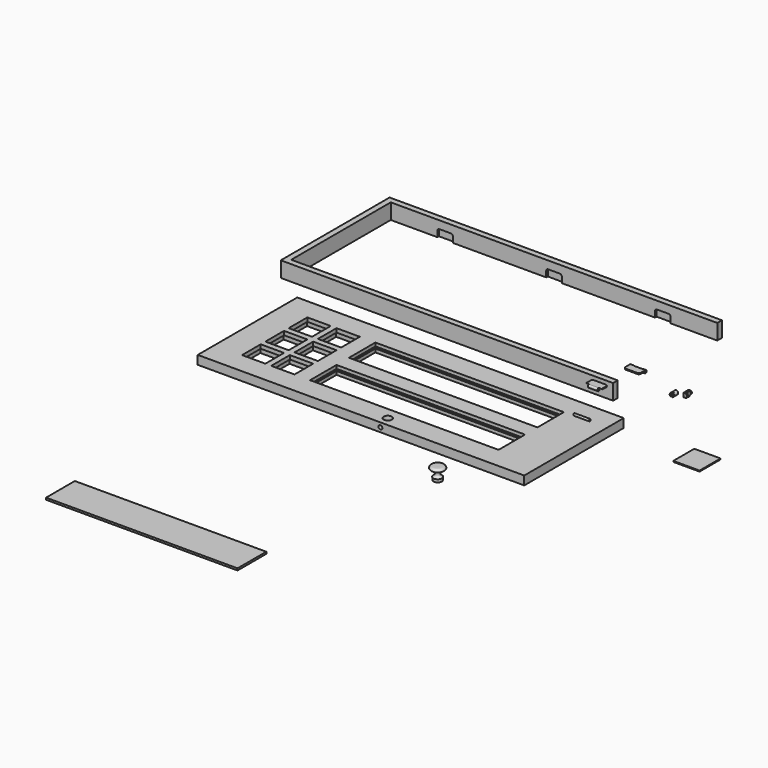
from build123d import *

# Parameters (mm, degrees)
F0_W      = 2133.6
F0_H      = 812.8
F0_W_2    = 152.4
F0_H_2    = 152.4
F0_W_3    = 1231.9
F0_H_3    = 215.9
F1_DEPTH  = 57.15
F2_R      = 6.985
F3_DEPTH  = 101.6
F6_DEPTH  = 63.5
F8_DEPTH  = 101.6
F10_R     = 9.525
F10_R_2   = 6.985
F11_DEPTH = 31.75
F12_R     = 6.985
F13_DEPTH = 101.6
F14_R     = 12.7
F14_2_R   = 12.7
F15_W     = 101.6
F15_H     = 50.8
F16_DEPTH = 6.35
F17_R     = 12.7
F19_DEPTH = 101.6
F20_W     = 101.6
F20_H     = 50.8
F21_DEPTH = 12.7
F22_R     = 12.7
F23_R     = 26.9875
F24_DEPTH = 393.7
F26_DEPTH = 57.658
F29_W     = 1250.95
F29_H     = 234.95
F29_W_2   = 1231.9
F29_H_2   = 215.9
F32_DEPTH = 12.7
F31_W     = 2.4516191959
F31_H     = 12.7
F31_W_2   = 9.525
F34_W     = 9.525
F34_H     = 12.7
F36_W     = 171.45
F36_H     = 171.45
F36_W_2   = 152.4
F36_H_2   = 152.4
F37_DEPTH = 31.75
F38_W     = 171.45
F38_H     = 171.45
F39_DEPTH = 6.35
F40_R     = 12.7
F41_DEPTH = 38.1
F42_W     = 12.7
F42_H     = 49.1664424331
F43_DEPTH = 12.7
F45_DEPTH = 39.624
F46_W     = 12.7
F46_H     = 25.4
F47_DEPTH = 50.8
F49_R     = 3.81
F50_DEPTH = 12.7
F51_R     = 12.69999
F52_W     = 9.8214453638
F52_H     = 25.4
F53_DEPTH = 6.35
F55_DEPTH = 12.7
F56_R     = 26.9875
F57_DEPTH = 19.05
F59_DEPTH = 12.7


# Not quite as in the source:
# - a fillet or chamfer is up to 0.001 mm smaller than in the source, because OpenCascade refuses the exact size


with BuildPart() as f1:
    # F0 (on Top) → F1 (new body)
    with BuildSketch(Plane.XY):
        with Locations((-1066.8, -406.4)):
            Rectangle(F0_W, F0_H)
        with Locations((-1879.6, -596.9)):
            Rectangle(F0_W_2, F0_H_2, mode=Mode.SUBTRACT)
        with Locations((-1689.1, -596.9)):
            Rectangle(F0_W_2, F0_H_2, mode=Mode.SUBTRACT)
        with Locations((-1879.6, -406.4)):
            Rectangle(F0_W_2, F0_H_2, mode=Mode.SUBTRACT)
        with Locations((-1689.1, -406.4)):
            Rectangle(F0_W_2, F0_H_2, mode=Mode.SUBTRACT)
        with Locations((-895.35, -565.15)):
            Rectangle(F0_W_3, F0_H_3, mode=Mode.SUBTRACT)
        with Locations((-1879.6, -215.9)):
            Rectangle(F0_W_2, F0_H_2, mode=Mode.SUBTRACT)
        with Locations((-1689.1, -215.9)):
            Rectangle(F0_W_2, F0_H_2, mode=Mode.SUBTRACT)
        with Locations((-895.35, -247.65)):
            Rectangle(F0_W_3, F0_H_3, mode=Mode.SUBTRACT)
    extrude(amount=F1_DEPTH)

    # F15 (on face) → F16 (cut)
    with BuildSketch(Plane(origin=(0, 0, 0), x_dir=(-1, 0, 0), z_dir=(0, 1, 0))):
        with Locations((355.6, 25.4)):
            Rectangle(F15_W, F15_H)
        with Locations((1778, 25.4)):
            Rectangle(F15_W, F15_H)
        with Locations((1066.8, 25.4)):
            Rectangle(F15_W, F15_H)
    extrude(amount=-F16_DEPTH, mode=Mode.SUBTRACT)

    # F17
    f17_edges = [f1.edges().sort_by_distance(p)[0] for p in [
        (-304.8, -3.175, 50.8),
        (-406.4, -3.175, 50.8),
        (-1117.6, -3.175, 50.8),
        (-1016, -3.175, 50.8),
        (-1727.2, -3.175, 50.8),
        (-1828.8, -3.175, 50.8),
    ]]
    fillet(f17_edges, radius=F17_R)

    # F23 (on face) → F24 (cut)
    with BuildSketch(Plane(origin=(0, 0, 0), x_dir=(1, 0, 0), z_dir=(0, 0, -1))):
        with Locations((-939.8, 752.475)):
            Circle(F23_R)
    extrude(amount=-F24_DEPTH, mode=Mode.SUBTRACT)

    # F25 (on face) → F26 (cut)
    with BuildSketch(Plane.XZ.offset(812.8)):
        with BuildLine():
            ThreePointArc((-952.5, 28.575), (-939.8, 15.875), (-927.1, 28.575))
            Line((-927.1, 28.575), (-952.5, 28.575))
        make_face()
        with BuildLine():
            Line((-952.5, 28.575), (-927.1, 28.575))
            ThreePointArc((-927.1, 28.575), (-939.8, 41.275), (-952.5, 28.575))
        make_face()
    extrude(amount=-F26_DEPTH, mode=Mode.SUBTRACT)

    # F33: sweep along a path in F33_path
    with BuildLine(Plane(origin=(-1511.3, -457.2, 0), x_dir=(0, 1, 0), z_dir=(0, 0, 1))) as f33_path:
        Line((0, 0), (0, -1231.9))
        Line((0, -1231.9), (-215.9, -1231.9))
        Line((-215.9, -1231.9), (-215.9, 0))
        Line((-215.9, 0), (0, 0))
    # F31 (on offset) → F33 (sweep, cut)
    with BuildSketch(Plane.YZ.offset(-627.38)):
        with Locations((-458.425809598, 28.575)):
            Rectangle(F31_W, F31_H)
        with Locations((-452.4375, 28.575)):
            Rectangle(F31_W_2, F31_H)
    sweep(path=f33_path.line, transition=Transition.RIGHT, mode=Mode.SUBTRACT)

    # F35: sweep along a path in F35_path
    with BuildLine(Plane(origin=(-279.4, -355.6, 0), x_dir=(0, 1, 0), z_dir=(0, 0, 1))) as f35_path:
        Line((0, 0), (0, 1231.9))
        Line((0, 1231.9), (215.9, 1231.9))
        Line((215.9, 1231.9), (215.9, 0))
        Line((215.9, 0), (0, 0))
    # F34 (on offset) → F35 (sweep, cut)
    with BuildSketch(Plane.YZ.offset(-627.38)):
        with Locations((-360.3625, 28.575)):
            Rectangle(F34_W, F34_H)
    sweep(path=f35_path.line, transition=Transition.RIGHT, mode=Mode.SUBTRACT)

    # F36 (on face) → F37 (cut)
    with BuildSketch(Plane(origin=(0, 0, 0), x_dir=(1, 0, 0), z_dir=(0, 0, -1))):
        with Locations((-1689.1, 596.9)):
            Rectangle(F36_W, F36_H)
        with Locations((-1689.1, 596.9)):
            Rectangle(F36_W_2, F36_H_2, mode=Mode.SUBTRACT)
        with Locations((-1879.6, 596.9)):
            Rectangle(F36_W, F36_H)
        with Locations((-1879.6, 596.9)):
            Rectangle(F36_W_2, F36_H_2, mode=Mode.SUBTRACT)
        with Locations((-1879.6, 406.4)):
            Rectangle(F36_W, F36_H)
        with Locations((-1879.6, 406.4)):
            Rectangle(F36_W_2, F36_H_2, mode=Mode.SUBTRACT)
        with Locations((-1689.1, 406.4)):
            Rectangle(F36_W, F36_H)
        with Locations((-1689.1, 406.4)):
            Rectangle(F36_W_2, F36_H_2, mode=Mode.SUBTRACT)
        with Locations((-1689.1, 215.9)):
            Rectangle(F36_W, F36_H)
        with Locations((-1689.1, 215.9)):
            Rectangle(F36_W_2, F36_H_2, mode=Mode.SUBTRACT)
        with Locations((-1879.6, 215.9)):
            Rectangle(F36_W, F36_H)
        with Locations((-1879.6, 215.9)):
            Rectangle(F36_W_2, F36_H_2, mode=Mode.SUBTRACT)
    extrude(amount=-F37_DEPTH, mode=Mode.SUBTRACT)


with BuildPart() as f3:
    # F2 (on Right) → F3 (new body)
    with BuildSketch(Plane.YZ):
        with BuildLine():
            Line((0, 339.3088579178), (41.8197438789, 339.3088579178))
            ThreePointArc((41.8197438789, 339.3088579178), (56.299261314, 328.3567279844), (50.8, 345.6588579178))
            Line((50.8, 345.6588579178), (0, 345.6588579178))
            Line((0, 345.6588579178), (0, 339.3088579178))
        make_face()
        with Locations((50.8, 336.1338579178)):
            Circle(F2_R, mode=Mode.SUBTRACT)
    extrude(amount=F3_DEPTH)

    # F5 (on offset) → F6 (cut)
    with BuildSketch(Plane.YZ.offset(82.55)):
        with BuildLine():
            ThreePointArc((50.8, 345.6588579178), (44.0648079092, 329.398665827), (60.325, 336.1338579178))
            ThreePointArc((60.325, 336.1338579178), (57.5351920908, 342.8690500086), (50.8, 345.6588579178))
        make_face()
    extrude(amount=-F6_DEPTH, mode=Mode.SUBTRACT)

    # F14#2
    f14_2_edges = [f3.edges().sort_by_distance(p)[0] for p in [
        (101.6, 0, 342.483858),
        (0, 0, 342.483858),
    ]]
    fillet(f14_2_edges, radius=F14_2_R)


with BuildPart() as f8:
    # F7 (on Right) → F8 (new body)
    with BuildSketch(Plane.YZ):
        with BuildLine():
            ThreePointArc((-181.1577074063, 298.6267453909), (-175.6584460923, 296.8788753242), (-172.1774512852, 292.2767453909))
            Line((-172.1774512852, 292.2767453909), (-130.3577074063, 292.2767453909))
            Line((-130.3577074063, 292.2767453909), (-130.3577074063, 298.6267453909))
            Line((-130.3577074063, 298.6267453909), (-181.1577074063, 298.6267453909))
        make_face()
    extrude(amount=-F8_DEPTH)

    # F10 (on offset) → F11 (join, symmetric)
    with BuildSketch(Plane.YZ.offset(-50.8)):
        with Locations((-181.1577074063, 289.1017453909)):
            Circle(F10_R)
        with Locations((-181.1577074063, 289.1017453909)):
            Circle(F10_R_2, mode=Mode.SUBTRACT)
    extrude(amount=F11_DEPTH, both=True)

    # F14
    f14_edges = [f8.edges().sort_by_distance(p)[0] for p in [
        (0, -130.357707, 295.451745),
        (-101.6, -130.357707, 295.451745),
    ]]
    fillet(f14_edges, radius=F14_R)


with BuildPart() as f13:
    # F12 (on Right) → F13 (new body)
    with BuildSketch(Plane.YZ):
        with Locations((-277.2486507893, 157.7363908291)):
            Circle(F12_R)
    extrude(amount=-F13_DEPTH)


with BuildPart() as f19:
    # F18 (on Top) → F19 (new body)
    with BuildSketch(Plane.XY):
        Polygon((-230.8065898895, 239.5188876568), (-2364.4065898895, 239.5188876568), (-2364.4065898895, 1052.3188876568), (-230.8065898895, 1052.3188876568), (-230.8065898895, 1090.4188876568), (-2402.5065898895, 1090.4188876568), (-2402.5065898895, 201.4188876568), (-230.8065898895, 201.4188876568), align=None)
    extrude(amount=F19_DEPTH)

    # F20 (on face) → F21 (cut)
    with BuildSketch(Plane.XZ.offset(-1052.3188876568)):
        with Locations((-2008.8065898895, 25.4)):
            Rectangle(F20_W, F20_H)
        with Locations((-586.4065898895, 25.4)):
            Rectangle(F20_W, F20_H)
        with Locations((-1297.6065898895, 25.4)):
            Rectangle(F20_W, F20_H)
    extrude(amount=-F21_DEPTH, mode=Mode.SUBTRACT)

    # F22
    f22_edges = [f19.edges().sort_by_distance(p)[0] for p in [
        (-1348.40659, 1058.668888, 50.8),
        (-1246.80659, 1058.668888, 50.8),
        (-1958.00659, 1058.668888, 50.8),
        (-2059.60659, 1058.668888, 50.8),
        (-637.20659, 1058.668888, 50.8),
        (-535.60659, 1058.668888, 50.8),
    ]]
    fillet(f22_edges, radius=F22_R)


with BuildPart() as f28:
    # F27 (on Right) → F28 (revolve)
    with BuildSketch(Plane.YZ):
        with BuildLine():
            Line((-1520.0962867782, 337.4846986438), (-1520.0962867782, 400.9846986438))
            add(Edge.make_bspline(
                [(-1520.0962867782, 400.9846986438), (-1534.2114565566, 401.6933648328), (-1554.579033096, 402.7159393447), (-1560.534572444, 398.1062998173), (-1566.8359177593, 389.1166628069), (-1559.9108352023, 381.6871503775), (-1550.2106903436, 377.7851827979), (-1536.7427785634, 380.346063669), (-1533.2248161057, 372.6538611018), (-1533.9660823746, 362.8511975489), (-1533.4473912198, 355.3453243062), (-1533.5099032617, 348.4605872031), (-1538.142814929, 344.899923605), (-1542.9701847467, 343.1729041488), (-1545.9344335349, 340.6946398649), (-1547.743199251, 338.5732138638), (-1548.6712867782, 337.4846986438)],
                knots=[0, 0, 0, 0, 0.1444656141, 0.2084576026, 0.2822883496, 0.3529619485, 0.4334819885, 0.5191310762, 0.5824060925, 0.6594691113, 0.7280822618, 0.7897608899, 0.8465830079, 0.90202106, 0.949726473, 1, 1, 1, 1], degree=3))
            Line((-1548.6712867782, 337.4846986438), (-1520.0962867782, 337.4846986438))
        make_face()
    revolve(axis=Axis((0, -1520.0962867782, 369.2346986438), (0, 0, -1)))

    # F56 (on face) → F57 (join)
    with BuildSketch(Plane(origin=(0, 0, 337.4846986438), x_dir=(1, 0, 0), z_dir=(0, 0, -1))):
        with Locations((0, 1520.0962867782)):
            Circle(F56_R)
    extrude(amount=F57_DEPTH)

    # F58 (on face) → F59 (cut)
    with BuildSketch(Plane(origin=(0, 0, 318.4346986438), x_dir=(1, 0, 0), z_dir=(0, 0, -1))):
        with BuildLine():
            ThreePointArc((3.7922780505, 1500.6894388013), (0, 1504.1323867782), (-3.7922780505, 1500.6894388013))
            ThreePointArc((-3.7922780505, 1500.6894388013), (0, 1500.3223867782), (3.7922780505, 1500.6894388013))
        make_face()
        with BuildLine():
            ThreePointArc((3.7922780505, 1500.6894388013), (0, 1500.3223867782), (-3.7922780505, 1500.6894388013))
            ThreePointArc((-3.7922780505, 1500.6894388013), (-0.1837397992, 1496.5168198446), (3.81, 1500.3223867782))
            ThreePointArc((3.81, 1500.3223867782), (3.8055669336, 1500.5061265773), (3.7922780505, 1500.6894388013))
        make_face()
    extrude(amount=-F59_DEPTH, mode=Mode.SUBTRACT)


with BuildPart() as f32:
    # F29 (on Top) → F32 (new body)
    with BuildSketch(Plane.XY):
        with Locations((-1180.55796282, -2343.5813390732)):
            Rectangle(F29_W, F29_H)
        with Locations((-1180.55796282, -2343.5813390732)):
            Rectangle(F29_W_2, F29_H_2, mode=Mode.SUBTRACT)
        with Locations((-1180.55796282, -2343.5813390732)):
            Rectangle(F29_W_2, F29_H_2)
    extrude(amount=F32_DEPTH)


with BuildPart() as f39:
    # F38 (on Top) → F39 (new body)
    with BuildSketch(Plane.XY):
        with Locations((517.6804175741, -49.3027456105)):
            Rectangle(F38_W, F38_H)
    extrude(amount=F39_DEPTH)


with BuildPart() as f41:
    # F40 (on Front) → F41 (new body)
    with BuildSketch(Plane.XZ):
        with Locations((343.2819247246, 316.3088858128)):
            Circle(F40_R)
    extrude(amount=F41_DEPTH)

    # F42 (on face) → F43 (cut)
    with BuildSketch(Plane.XZ.offset(38.1)):
        with Locations((343.2819247246, 316.3088858128)):
            Rectangle(F42_W, F42_H)
    extrude(amount=-F43_DEPTH, mode=Mode.SUBTRACT)

    # F44 (on face) → F45 (cut, symmetric)
    with BuildSketch(Plane.YZ.offset(336.9319247246)):
        with BuildLine():
            ThreePointArc((-27.94, 316.3088858128), (-29.0559231637, 319.0029626491), (-31.75, 320.1188858128))
            Line((-31.75, 320.1188858128), (-31.75, 312.4988858128))
            ThreePointArc((-31.75, 312.4988858128), (-29.0559231637, 313.6148089764), (-27.94, 316.3088858128))
        make_face()
        with BuildLine():
            Line((-31.75, 312.4988858128), (-31.75, 320.1188858128))
            ThreePointArc((-31.75, 320.1188858128), (-35.56, 316.3088858128), (-31.75, 312.4988858128))
        make_face()
    extrude(amount=F45_DEPTH, both=True, mode=Mode.SUBTRACT)


with BuildPart() as f47:
    # F46 (on Front) → F47 (new body)
    with BuildSketch(Plane.XZ):
        with Locations((437.0324688339, 350.949629081)):
            Rectangle(F46_W, F46_H)
    extrude(amount=F47_DEPTH)

    # F49 (on offset) → F50 (join, symmetric)
    with BuildSketch(Plane.YZ.offset(437.0324688339)):
        with Locations((-6.35, 350.949629081)):
            Circle(F49_R)
    extrude(amount=F50_DEPTH, both=True)

    # F51 (radius 12.7 in the source; OpenCascade refuses exactly that, so slightly less here)
    f51_edges = [f47.edges().sort_by_distance(p)[0] for p in [
        (437.032469, 0, 363.649629),
        (437.032469, 0, 338.249629),
    ]]
    fillet(f51_edges, radius=F51_R)

    # F52 (on face) → F53 (join)
    with BuildSketch(Plane.YZ.offset(443.3824688339)):
        with Locations((-45.8892773181, 350.949629081)):
            Rectangle(F52_W, F52_H)
    extrude(amount=F53_DEPTH)

    # F54 (on face) → F55 (join)
    with BuildSketch(Plane.YZ.offset(449.7324688339)):
        with BuildLine():
            ThreePointArc((-42.0792773181, 350.949629081), (-43.1952004818, 353.6437059173), (-45.8892773181, 354.759629081))
            Line((-45.8892773181, 354.759629081), (-45.8892773181, 347.139629081))
            ThreePointArc((-45.8892773181, 347.139629081), (-43.1952004818, 348.2555522447), (-42.0792773181, 350.949629081))
        make_face()
        with BuildLine():
            Line((-45.8892773181, 347.139629081), (-45.8892773181, 354.759629081))
            ThreePointArc((-45.8892773181, 354.759629081), (-49.6992773181, 350.949629081), (-45.8892773181, 347.139629081))
        make_face()
    extrude(amount=F55_DEPTH)


solid = Compound([f1.part, f3.part, f8.part, f13.part, f19.part, f28.part, f32.part, f39.part, f41.part, f47.part])
